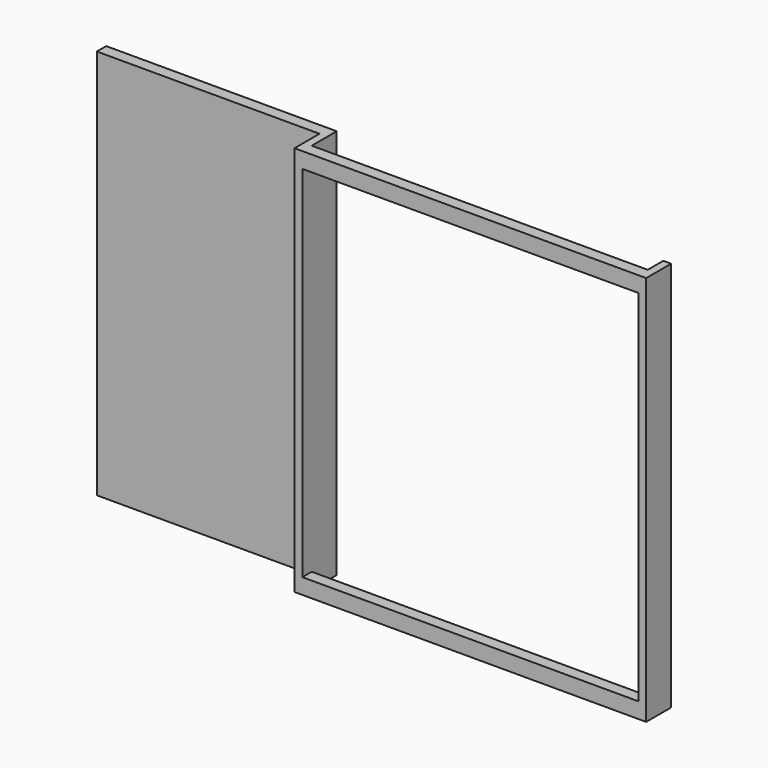
from build123d import *

# Parameters (mm, degrees)
F2_DEPTH = 100
F3_W     = 86
F3_H     = 92
F4_DEPTH = 3


# Not quite as in the source:
# - the program builds the solid bodies; features that only make, move or delete a surface that nothing else refers to are left out


with BuildPart() as f2:
    # F0 (on Top) → F2 (new body)
    with BuildSketch(Plane.XY):
        Polygon((-2.3052925244, 0), (87.6947074756, 0), (87.6947074756, 8), (85.6947074756, 8), (85.6947074756, 3), (-0.3052925244, 3), (-0.3052925244, 11), (-59.3052925244, 11), (-59.3052925244, 8), (-2.3052925244, 8), (-2.3052925244, 3), align=None)
    extrude(amount=-F2_DEPTH)

    # F3 (on Front) → F4 (cut)
    with BuildSketch(Plane.XZ):
        with Locations((42.6947074756, -50)):
            Rectangle(F3_W, F3_H)
    extrude(amount=-F4_DEPTH, mode=Mode.SUBTRACT)


solid = f2.part
